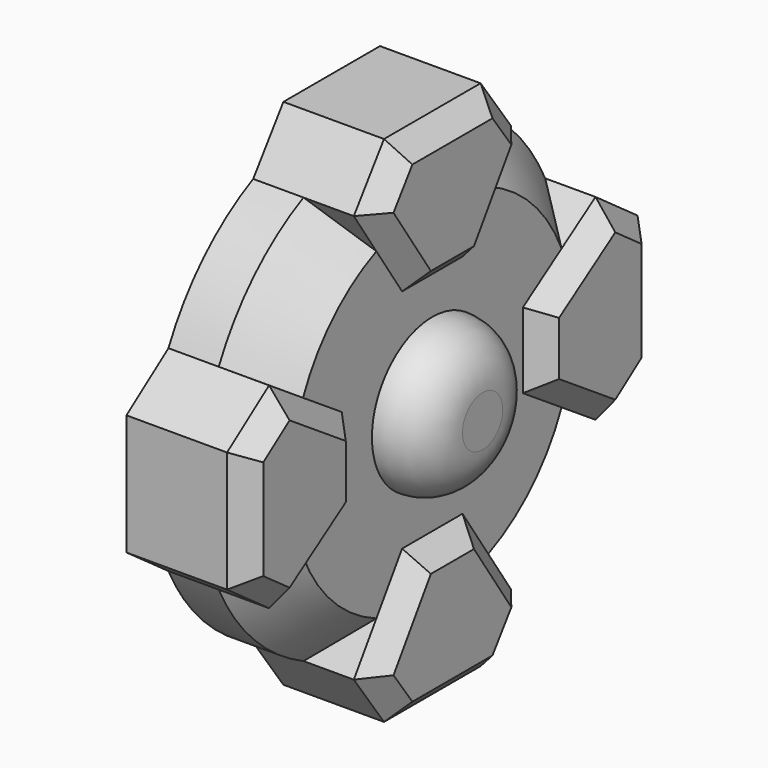
from build123d import *

# Parameters (mm, degrees)
F1_DEPTH = 10
F2_DEPTH = 12
F3_SIZE  = 5
F4_SIZE  = 1.99999
F5_R     = 7.5
F6_DEPTH = 5
F7_R     = 4.99999
F9_DEPTH = 3


# Not quite as in the source:
# - a fillet or chamfer is up to 0.001 mm smaller than in the source, because OpenCascade refuses the exact size
# - a feature names something its author has since deleted; it is built from what else it names


with BuildPart() as f1:
    # F0 (on Right) → F1 (new body)
    with BuildSketch(Plane.YZ):
        with BuildLine():
            Line((11.25, 3.75), (20.2777587519, 9.75))
            ThreePointArc((20.2777587519, 9.75), (15.9099025767, 15.9099025767), (9.75, 20.2777587519))
            Line((9.75, 20.2777587519), (3.75, 11.25))
            Line((3.75, 11.25), (0, 11.25))
            Line((0, 11.25), (-3.75, 11.25))
            Line((-3.75, 11.25), (-9.75, 20.2777587519))
            ThreePointArc((-9.75, 20.2777587519), (-15.9099025767, 15.9099025767), (-20.2777587519, 9.75))
            Line((-20.2777587519, 9.75), (-11.25, 3.75))
            Line((-11.25, 3.75), (-11.25, 0))
            Line((-11.25, 0), (-11.25, -3.75))
            Line((-11.25, -3.75), (-20.2777587519, -9.75))
            ThreePointArc((-20.2777587519, -9.75), (-15.9099025767, -15.9099025767), (-9.75, -20.2777587519))
            Line((-9.75, -20.2777587519), (-3.75, -11.25))
            Line((-3.75, -11.25), (0, -11.25))
            Line((0, -11.25), (3.75, -11.25))
            Line((3.75, -11.25), (9.75, -20.2777587519))
            ThreePointArc((9.75, -20.2777587519), (15.9099025767, -15.9099025767), (20.2777587519, -9.75))
            Line((20.2777587519, -9.75), (11.25, -3.75))
            Line((11.25, -3.75), (11.25, 0))
            Line((11.25, 0), (11.25, 3.75))
        make_face()
    extrude(amount=F1_DEPTH)

    # F0 (on Right) → F2 (join)
    with BuildSketch(Plane.YZ):
        with BuildLine():
            Line((3.75, 11.25), (9.75, 20.2777587519))
            ThreePointArc((9.75, 20.2777587519), (0, 22.5), (-9.75, 20.2777587519))
            Line((-9.75, 20.2777587519), (-3.75, 11.25))
            Line((-3.75, 11.25), (0, 11.25))
            Line((0, 11.25), (3.75, 11.25))
        make_face()
        with BuildLine():
            ThreePointArc((-9.75, 20.2777587519), (0, 22.5), (9.75, 20.2777587519))
            Line((9.75, 20.2777587519), (6, 25.5))
            Line((6, 25.5), (0, 25.5))
            Line((0, 25.5), (-6, 25.5))
            Line((-6, 25.5), (-9.75, 20.2777587519))
        make_face()
        with BuildLine():
            Line((-11.25, 3.75), (-20.2777587519, 9.75))
            ThreePointArc((-20.2777587519, 9.75), (-22.5, 0), (-20.2777587519, -9.75))
            Line((-20.2777587519, -9.75), (-11.25, -3.75))
            Line((-11.25, -3.75), (-11.25, 0))
            Line((-11.25, 0), (-11.25, 3.75))
        make_face()
        with BuildLine():
            ThreePointArc((-20.2777587519, -9.75), (-22.5, 0), (-20.2777587519, 9.75))
            Line((-20.2777587519, 9.75), (-25.5, 6))
            Line((-25.5, 6), (-25.5, 0))
            Line((-25.5, 0), (-25.5, -6))
            Line((-25.5, -6), (-20.2777587519, -9.75))
        make_face()
        with BuildLine():
            ThreePointArc((-9.75, -20.2777587519), (0, -22.5), (9.75, -20.2777587519))
            Line((9.75, -20.2777587519), (3.75, -11.25))
            Line((3.75, -11.25), (0, -11.25))
            Line((0, -11.25), (-3.75, -11.25))
            Line((-3.75, -11.25), (-9.75, -20.2777587519))
        make_face()
        with BuildLine():
            Line((6, -25.5), (9.75, -20.2777587519))
            ThreePointArc((9.75, -20.2777587519), (0, -22.5), (-9.75, -20.2777587519))
            Line((-9.75, -20.2777587519), (-6, -25.5))
            Line((-6, -25.5), (0, -25.5))
            Line((0, -25.5), (6, -25.5))
        make_face()
        with BuildLine():
            ThreePointArc((20.2777587519, -9.75), (21.93740609, -5.0000214041), (22.5, 0))
            ThreePointArc((22.5, 0), (21.93740609, 5.0000214041), (20.2777587519, 9.75))
            Line((20.2777587519, 9.75), (11.25, 3.75))
            Line((11.25, 3.75), (11.25, 0))
            Line((11.25, 0), (11.25, -3.75))
            Line((11.25, -3.75), (20.2777587519, -9.75))
        make_face()
        with BuildLine():
            ThreePointArc((20.2777587519, 9.75), (21.93740609, 5.0000214041), (22.5, 0))
            ThreePointArc((22.5, 0), (21.93740609, -5.0000214041), (20.2777587519, -9.75))
            Line((20.2777587519, -9.75), (25.5, -6))
            Line((25.5, -6), (25.5, 0))
            Line((25.5, 0), (25.5, 6))
            Line((25.5, 6), (20.2777587519, 9.75))
        make_face()
    extrude(amount=F2_DEPTH)

    # F3
    f3_edges = [f1.edges().sort_by_distance(p)[0] for p in [
        (10, 15.909903, 15.909903),
        (10, -15.909903, 15.909903),
        (10, -15.909903, -15.909903),
        (10, 15.909903, -15.909903),
    ]]
    chamfer(f3_edges, length=F3_SIZE)

    # F4 (size 2 in the source; OpenCascade refuses exactly that, so slightly less here)
    f4_edges = [f1.edges().sort_by_distance(p)[0] for p in [
        (12, 0, 25.5),
        (12, -7.875, 22.888879),
        (12, 7.875, 22.888879),
        (12, -6.75, 15.763879),
        (12, 6.75, 15.763879),
        (12, 0, 11.25),
        (12, -15.763879, 6.75),
        (12, -22.888879, 7.875),
        (12, -25.5, 0),
        (12, -22.888879, -7.875),
        (12, -15.763879, -6.75),
        (12, -11.25, 0),
        (12, 0, -11.25),
        (12, -6.75, -15.763879),
        (12, -7.875, -22.888879),
        (12, 6.75, -15.763879),
        (12, 0, -25.5),
        (12, 7.875, -22.888879),
        (12, 15.763879, -6.75),
        (12, 11.25, 0),
        (12, 15.763879, 6.75),
        (12, 22.888879, 7.875),
        (12, 25.5, 0),
        (12, 22.888879, -7.875),
    ]]
    chamfer(f4_edges, length=F4_SIZE)

    # F5 (on face) → F6 (join)
    with BuildSketch(Plane.YZ.offset(10)):
        Circle(F5_R)
    extrude(amount=F6_DEPTH)

    # F7 (radius 5 in the source; OpenCascade refuses exactly that, so slightly less here)
    f7_edges = [f1.edges().sort_by_distance(p)[0] for p in [
        (15, -7.5, 0),
    ]]
    fillet(f7_edges, radius=F7_R)

    # F8 (on face) → F9 (cut)
    with BuildSketch(Plane.YZ):
        with BuildLine():
            ThreePointArc((0, -11.25), (7.9549512883, -7.9549512883), (11.25, 0))
            ThreePointArc((11.25, 0), (7.9549512883, 7.9549512883), (0, 11.25))
            ThreePointArc((0, 11.25), (-7.9549512883, 7.9549512883), (-11.25, 0))
            ThreePointArc((-11.25, 0), (-7.9549512883, -7.9549512883), (0, -11.25))
        make_face()
    extrude(amount=F9_DEPTH, mode=Mode.SUBTRACT)


solid = f1.part
